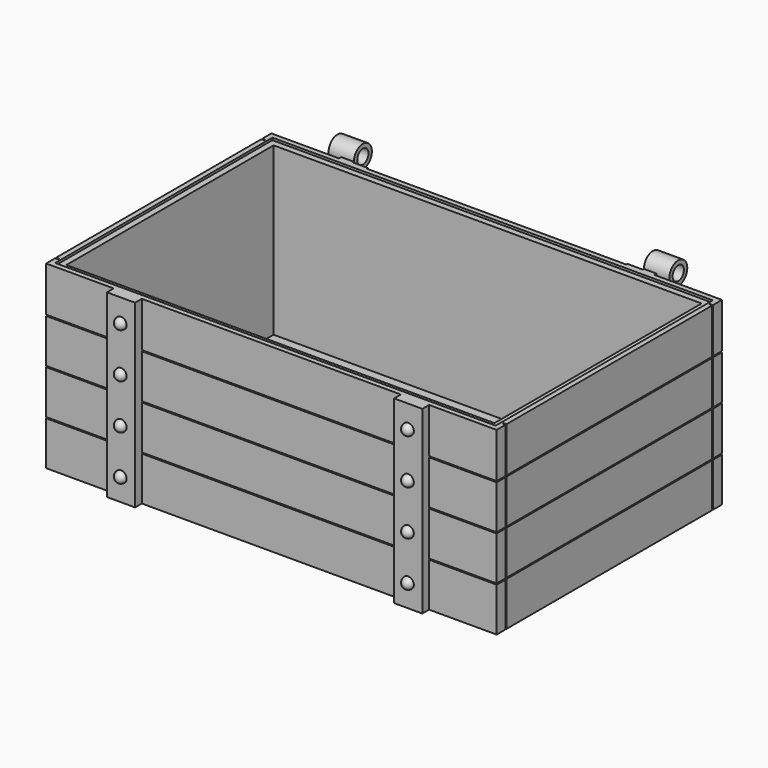
from build123d import *

# Parameters (mm, degrees)
F0_W      = 80
F0_H      = 50
F1_DEPTH  = 2
F2_W      = 80
F2_H      = 50
F2_W_2    = 76
F2_H_2    = 46
F3_DEPTH  = 30
F4_W      = 5
F4_H      = 32
F5_DEPTH  = 1.5
F6_R      = 2
F7_DEPTH  = 2.25
F8_R      = 2
F9_DEPTH  = 2.25
F10_R     = 1.25
F11_DEPTH = 35
F12_W     = 5
F12_H     = 32
F13_DEPTH = 1.5
F15_DEPTH = 2.75
F17_DEPTH = 2.75
F18_R     = 1
F19_R     = 1
F20_DEPTH = 1
F21_R     = 0.99999
F22_R     = 1
F23_R     = 1
F24_DEPTH = 1
F25_R     = 0.99999
F26_W     = 12
F26_H     = 0.2
F26_W_2   = 46
F27_DEPTH = 0.5
F28_W     = 12
F28_H     = 0.2
F28_W_2   = 46
F29_DEPTH = 0.5
F30_W     = 0.2
F30_H     = 8
F30_H_2   = 0.2
F30_W_2   = 2
F30_W_3   = 45.6
F30_H_3   = 7.8
F31_DEPTH = 0.5
F32_W     = 0.2
F32_H     = 8
F32_H_2   = 0.2
F32_W_2   = 2
F32_W_3   = 45.6
F32_H_3   = 7.8
F33_DEPTH = 0.5
F34_W     = 78.2
F34_H     = 48.2
F34_W_2   = 76
F34_H_2   = 46
F35_DEPTH = 0.4


# Not quite as in the source:
# - a fillet or chamfer is up to 0.001 mm smaller than in the source, because OpenCascade refuses the exact size


with BuildPart() as f1:
    # F0 (on Top) → F1 (new body)
    with BuildSketch(Plane.XY):
        Rectangle(F0_W, F0_H)
    extrude(amount=F1_DEPTH)

    # F2 (on face) → F3 (join)
    with BuildSketch(Plane.XY.offset(2)):
        Rectangle(F2_W, F2_H)
        Rectangle(F2_W_2, F2_H_2, mode=Mode.SUBTRACT)
    extrude(amount=F3_DEPTH)

    # F4 (on face) → F5 (join)
    with BuildSketch(Plane(origin=(0, 25, 0), x_dir=(-1, 0, 0), z_dir=(0, 1, 0))):
        with Locations((-25.5, 16)):
            Rectangle(F4_W, F4_H)
        with Locations((25.5, 16)):
            Rectangle(F4_W, F4_H)
    extrude(amount=F5_DEPTH)

    # F6 (on face) → F7 (join, symmetric)
    with BuildSketch(Plane.YZ.offset(28)):
        with Locations((27.5, 32)):
            Circle(F6_R)
    extrude(amount=F7_DEPTH, both=True)

    # F8 (on face) → F9 (join, symmetric)
    with BuildSketch(Plane(origin=(-28, 0, 0), x_dir=(0, -1, 0), z_dir=(-1, 0, 0))):
        with Locations((-27.5, 32)):
            Circle(F8_R)
    extrude(amount=F9_DEPTH, both=True)

    # F10 (on Right) → F11 (cut, symmetric)
    with BuildSketch(Plane.YZ):
        with Locations((27.5, 32)):
            Circle(F10_R)
    extrude(amount=F11_DEPTH, both=True, mode=Mode.SUBTRACT)

    # F12 (on face) → F13 (join)
    with BuildSketch(Plane.XZ.offset(25)):
        with Locations((-25.5, 16)):
            Rectangle(F12_W, F12_H)
        with Locations((25.5, 16)):
            Rectangle(F12_W, F12_H)
    extrude(amount=F13_DEPTH)

    # F14 (on face) → F15 (cut, through all)
    with BuildSketch(Plane.YZ.offset(-23)):
        with BuildLine():
            Line((26.25, 32), (25.25, 32))
            ThreePointArc((25.25, 32), (25.5878676824, 30.8141458774), (26.5, 29.9844355629))
            Line((26.5, 29.9844355629), (26.5, 31.25))
            ThreePointArc((26.5, 31.25), (26.3141458774, 31.6047152925), (26.25, 32))
        make_face()
    extrude(amount=-F15_DEPTH, mode=Mode.SUBTRACT)

    # F16 (on face) → F17 (cut, through all)
    with BuildSketch(Plane(origin=(23, 0, 0), x_dir=(0, -1, 0), z_dir=(-1, 0, 0))):
        with BuildLine():
            Line((-26.25, 32), (-25.25, 32))
            ThreePointArc((-25.25, 32), (-29.4121323176, 33.1858541226), (-26.5, 29.9844355629))
            Line((-26.5, 29.9844355629), (-26.5, 31.25))
            ThreePointArc((-26.5, 31.25), (-26.3141458774, 31.6047152925), (-26.25, 32))
        make_face()
        with BuildLine():
            ThreePointArc((-26.5, 29.9844355629), (-25.5878676824, 30.8141458774), (-25.25, 32))
            Line((-25.25, 32), (-26.25, 32))
            ThreePointArc((-26.25, 32), (-26.3141458774, 31.6047152925), (-26.5, 31.25))
            Line((-26.5, 31.25), (-26.5, 29.9844355629))
        make_face()
    extrude(amount=-F17_DEPTH, mode=Mode.SUBTRACT)

    # F18 (on face) + F19 (on face) → F20 (join)
    with BuildSketch(Plane.XZ.offset(26.5)):
        with Locations((-25.5, 28)):
            Circle(F18_R)
        with Locations((-25.5, 20)):
            Circle(F18_R)
        with Locations((-25.5, 12)):
            Circle(F18_R)
        with Locations((-25.5, 4)):
            Circle(F18_R)
    with BuildSketch(Plane.XZ.offset(26.5)):
        with Locations((25.5, 28)):
            Circle(F19_R)
        with Locations((25.5, 20)):
            Circle(F19_R)
        with Locations((25.5, 12)):
            Circle(F19_R)
        with Locations((25.5, 4)):
            Circle(F19_R)
    extrude(amount=F20_DEPTH)

    # F21 (radius 1 in the source; OpenCascade refuses exactly that, so slightly less here)
    f21_edges = [f1.edges().sort_by_distance(p)[0] for p in [
        (-26.5, -27.5, 28),
        (-26.5, -27.5, 20),
        (-26.5, -27.5, 12),
        (-26.5, -27.5, 4),
        (24.5, -27.5, 28),
        (24.5, -27.5, 20),
        (24.5, -27.5, 12),
        (24.5, -27.5, 4),
    ]]
    fillet(f21_edges, radius=F21_R)

    # F22 (on face) + F23 (on face) → F24 (join)
    with BuildSketch(Plane(origin=(0, 26.5, 0), x_dir=(-1, 0, 0), z_dir=(0, 1, 0))):
        with Locations((-25.5, 28)):
            Circle(F22_R)
        with Locations((-25.5, 20)):
            Circle(F22_R)
        with Locations((-25.5, 12)):
            Circle(F22_R)
        with Locations((-25.5, 4)):
            Circle(F22_R)
    with BuildSketch(Plane(origin=(0, 26.5, 0), x_dir=(-1, 0, 0), z_dir=(0, 1, 0))):
        with Locations((25.5, 28)):
            Circle(F23_R)
        with Locations((25.5, 20)):
            Circle(F23_R)
        with Locations((25.5, 12)):
            Circle(F23_R)
        with Locations((25.5, 4)):
            Circle(F23_R)
    extrude(amount=F24_DEPTH)

    # F25 (radius 1 in the source; OpenCascade refuses exactly that, so slightly less here)
    f25_edges = [f1.edges().sort_by_distance(p)[0] for p in [
        (26.5, 27.5, 28),
        (26.5, 27.5, 20),
        (26.5, 27.5, 12),
        (26.5, 27.5, 4),
        (-24.5, 27.5, 28),
        (-24.5, 27.5, 20),
        (-24.5, 27.5, 12),
        (-24.5, 27.5, 4),
    ]]
    fillet(f25_edges, radius=F25_R)

    # F26 (on face) → F27 (cut)
    with BuildSketch(Plane.XZ.offset(25)):
        with Locations((-34, 23.9)):
            Rectangle(F26_W, F26_H)
        with Locations((-34, 15.9)):
            Rectangle(F26_W, F26_H)
        with Locations((-34, 7.9)):
            Rectangle(F26_W, F26_H)
        with Locations((0, 7.9)):
            Rectangle(F26_W_2, F26_H)
        with Locations((0, 15.9)):
            Rectangle(F26_W_2, F26_H)
        with Locations((0, 23.9)):
            Rectangle(F26_W_2, F26_H)
        with Locations((34, 23.9)):
            Rectangle(F26_W, F26_H)
        with Locations((34, 15.9)):
            Rectangle(F26_W, F26_H)
        with Locations((34, 7.9)):
            Rectangle(F26_W, F26_H)
    extrude(amount=-F27_DEPTH, mode=Mode.SUBTRACT)

    # F28 (on face) → F29 (cut)
    with BuildSketch(Plane(origin=(0, 25, 0), x_dir=(-1, 0, 0), z_dir=(0, 1, 0))):
        with Locations((-34, 23.9)):
            Rectangle(F28_W, F28_H)
        with Locations((-34, 15.9)):
            Rectangle(F28_W, F28_H)
        with Locations((-34, 7.9)):
            Rectangle(F28_W, F28_H)
        with Locations((0, 23.9)):
            Rectangle(F28_W_2, F28_H)
        with Locations((0, 15.9)):
            Rectangle(F28_W_2, F28_H)
        with Locations((0, 7.9)):
            Rectangle(F28_W_2, F28_H)
        with Locations((34, 23.9)):
            Rectangle(F28_W, F28_H)
        with Locations((34, 15.9)):
            Rectangle(F28_W, F28_H)
        with Locations((34, 7.9)):
            Rectangle(F28_W, F28_H)
    extrude(amount=-F29_DEPTH, mode=Mode.SUBTRACT)

    # F30 (on face) → F31 (cut)
    with BuildSketch(Plane.YZ.offset(40)):
        with Locations((-22.9, 28)):
            Rectangle(F30_W, F30_H)
        with Locations((-22.9, 23.9)):
            Rectangle(F30_W, F30_H_2)
        with Locations((-24, 23.9)):
            Rectangle(F30_W_2, F30_H_2)
        with Locations((0, 23.9)):
            Rectangle(F30_W_3, F30_H_2)
        with Locations((-22.9, 19.9)):
            Rectangle(F30_W, F30_H_3)
        with Locations((22.9, 23.9)):
            Rectangle(F30_W, F30_H_2)
        with Locations((22.9, 28)):
            Rectangle(F30_W, F30_H)
        with Locations((-22.9, 15.9)):
            Rectangle(F30_W, F30_H_2)
        with Locations((-24, 15.9)):
            Rectangle(F30_W_2, F30_H_2)
        with Locations((22.9, 19.9)):
            Rectangle(F30_W, F30_H_3)
        with Locations((24, 23.9)):
            Rectangle(F30_W_2, F30_H_2)
        with Locations((-22.9, 11.9)):
            Rectangle(F30_W, F30_H_3)
        with Locations((22.9, 15.9)):
            Rectangle(F30_W, F30_H_2)
        with Locations((-22.9, 7.9)):
            Rectangle(F30_W, F30_H_2)
        with Locations((-24, 7.9)):
            Rectangle(F30_W_2, F30_H_2)
        with Locations((0, 7.9)):
            Rectangle(F30_W_3, F30_H_2)
        with Locations((22.9, 11.9)):
            Rectangle(F30_W, F30_H_3)
        with Locations((24, 15.9)):
            Rectangle(F30_W_2, F30_H_2)
        with Locations((-22.9, 3.9)):
            Rectangle(F30_W, F30_H_3)
        with Locations((22.9, 7.9)):
            Rectangle(F30_W, F30_H_2)
        with Locations((22.9, 3.9)):
            Rectangle(F30_W, F30_H_3)
        with Locations((24, 7.9)):
            Rectangle(F30_W_2, F30_H_2)
        with Locations((0, 15.9)):
            Rectangle(F30_W_3, F30_H_2)
    extrude(amount=-F31_DEPTH, mode=Mode.SUBTRACT)

    # F32 (on face) → F33 (cut)
    with BuildSketch(Plane(origin=(-40, 0, 0), x_dir=(0, -1, 0), z_dir=(-1, 0, 0))):
        with Locations((-22.9, 28)):
            Rectangle(F32_W, F32_H)
        with Locations((-22.9, 23.9)):
            Rectangle(F32_W, F32_H_2)
        with Locations((-24, 23.9)):
            Rectangle(F32_W_2, F32_H_2)
        with Locations((0, 23.9)):
            Rectangle(F32_W_3, F32_H_2)
        with Locations((-22.9, 19.9)):
            Rectangle(F32_W, F32_H_3)
        with Locations((22.9, 23.9)):
            Rectangle(F32_W, F32_H_2)
        with Locations((22.9, 28)):
            Rectangle(F32_W, F32_H)
        with Locations((-22.9, 15.9)):
            Rectangle(F32_W, F32_H_2)
        with Locations((-24, 15.9)):
            Rectangle(F32_W_2, F32_H_2)
        with Locations((22.9, 19.9)):
            Rectangle(F32_W, F32_H_3)
        with Locations((24, 23.9)):
            Rectangle(F32_W_2, F32_H_2)
        with Locations((-22.9, 11.9)):
            Rectangle(F32_W, F32_H_3)
        with Locations((22.9, 15.9)):
            Rectangle(F32_W, F32_H_2)
        with Locations((-22.9, 7.9)):
            Rectangle(F32_W, F32_H_2)
        with Locations((-24, 7.9)):
            Rectangle(F32_W_2, F32_H_2)
        with Locations((0, 7.9)):
            Rectangle(F32_W_3, F32_H_2)
        with Locations((22.9, 11.9)):
            Rectangle(F32_W, F32_H_3)
        with Locations((24, 15.9)):
            Rectangle(F32_W_2, F32_H_2)
        with Locations((-22.9, 3.9)):
            Rectangle(F32_W, F32_H_3)
        with Locations((22.9, 7.9)):
            Rectangle(F32_W, F32_H_2)
        with Locations((22.9, 3.9)):
            Rectangle(F32_W, F32_H_3)
        with Locations((24, 7.9)):
            Rectangle(F32_W_2, F32_H_2)
        with Locations((0, 15.9)):
            Rectangle(F32_W_3, F32_H_2)
    extrude(amount=-F33_DEPTH, mode=Mode.SUBTRACT)

    # F34 (on face) → F35 (cut)
    with BuildSketch(Plane.XY.offset(32)):
        Rectangle(F34_W, F34_H)
        Rectangle(F34_W_2, F34_H_2, mode=Mode.SUBTRACT)
    extrude(amount=-F35_DEPTH, mode=Mode.SUBTRACT)


solid = f1.part
